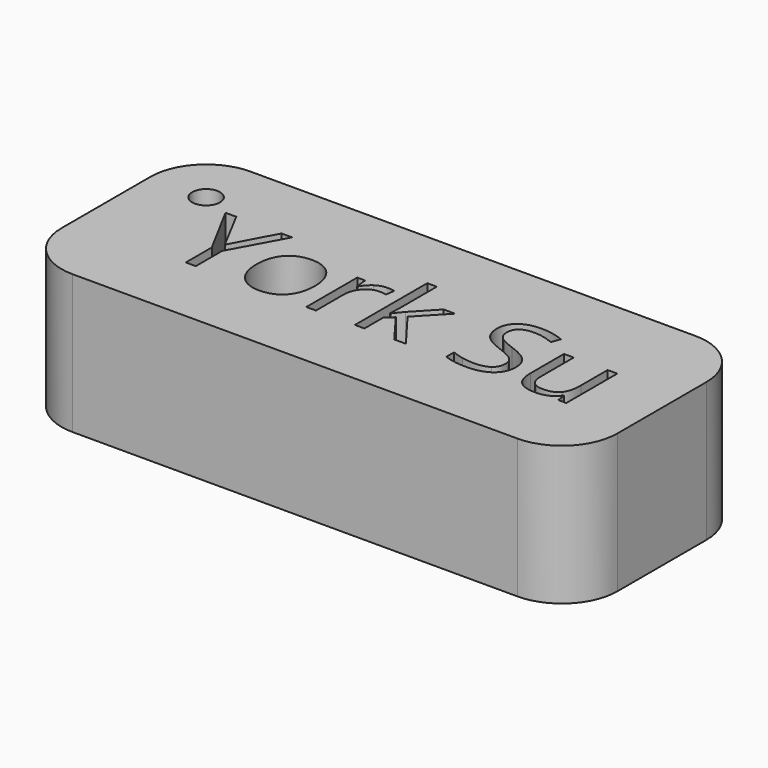
from build123d import *

# Parameters (mm, degrees)
F0_R     = 2.5
F1_DEPTH = 25


with BuildPart() as f1:
    # F0 (on Top) → F1 (new body)
    with BuildSketch(Plane.XY):
        with BuildLine():
            Line((90, 37.539282998), (10, 37.539282998))
            ThreePointArc((10, 37.539282998), (2.9289321881, 34.6103508099), (0, 27.539282998))
            Line((0, 27.539282998), (0, 7.539282998))
            ThreePointArc((0, 7.539282998), (2.9289321881, 0.4682151861), (10, -2.460717002))
            Line((10, -2.460717002), (90, -2.460717002))
            ThreePointArc((90, -2.460717002), (97.0710678119, 0.4682151861), (100, 7.539282998))
            Line((100, 7.539282998), (100, 27.539282998))
            ThreePointArc((100, 27.539282998), (97.0710678119, 34.6103508099), (90, 37.539282998))
        make_face()
        with BuildLine():
            add(Edge.make_bspline(
                [(37.3762699946, 20.3398448807), (38.7935582809, 18.7384931806), (38.7935582809, 16.0110080489)],
                knots=[0, 0, 0, 1, 1, 1], degree=2))
            add(Edge.make_bspline(
                [(38.7935582809, 16.0110080489), (38.7935582809, 13.2065509441), (37.3829632097, 11.6319721042)],
                knots=[0, 0, 0, 1, 1, 1], degree=2))
            add(Edge.make_bspline(
                [(37.3829632097, 11.6319721042), (35.9723681385, 10.0573932643), (33.4824921409, 10.0573932643)],
                knots=[0, 0, 0, 1, 1, 1], degree=2))
            add(Edge.make_bspline(
                [(33.4824921409, 10.0573932643), (31.94305268, 10.0573932643), (30.7516604016, 10.7802604894)],
                knots=[0, 0, 0, 1, 1, 1], degree=2))
            add(Edge.make_bspline(
                [(30.7516604016, 10.7802604894), (29.5602681232, 11.5031277145), (28.9110262636, 12.8518105466)],
                knots=[0, 0, 0, 1, 1, 1], degree=2))
            add(Edge.make_bspline(
                [(28.9110262636, 12.8518105466), (28.261784404, 14.2004933786), (28.261784404, 16.0110080489)],
                knots=[0, 0, 0, 1, 1, 1], degree=2))
            add(Edge.make_bspline(
                [(28.261784404, 16.0110080489), (28.261784404, 18.8121185462), (29.6640129564, 20.3766575635)],
                knots=[0, 0, 0, 1, 1, 1], degree=2))
            add(Edge.make_bspline(
                [(29.6640129564, 20.3766575635), (31.0662415088, 21.9411965808), (33.5561175064, 21.9411965808)],
                knots=[0, 0, 0, 1, 1, 1], degree=2))
            add(Edge.make_bspline(
                [(33.5561175064, 21.9411965808), (35.9589817084, 21.9411965808), (37.3762699946, 20.3398448807)],
                knots=[0, 0, 0, 1, 1, 1], degree=2))
        make_face(mode=Mode.SUBTRACT)
        with BuildLine():
            add(Edge.make_bspline(
                [(45.0918736404, 21.3337873152), (45.9921110642, 21.9411965808), (47.0697186868, 21.9411965808)],
                knots=[0, 0, 0, 1, 1, 1], degree=2))
            add(Edge.make_bspline(
                [(47.0697186868, 21.9411965808), (47.8327452022, 21.9411965808), (48.438481164, 21.8140254949)],
                knots=[0, 0, 0, 1, 1, 1], degree=2))
            Line((48.438481164, 21.8140254949), (48.1975254223, 20.204307276))
            add(Edge.make_bspline(
                [(48.1975254223, 20.204307276), (47.4880446273, 20.3615978296), (46.9425476009, 20.3615978296)],
                knots=[0, 0, 0, 1, 1, 1], degree=2))
            add(Edge.make_bspline(
                [(46.9425476009, 20.3615978296), (45.5503588711, 20.3615978296), (44.5631096516, 19.2321177904)],
                knots=[0, 0, 0, 1, 1, 1], degree=2))
            add(Edge.make_bspline(
                [(44.5631096516, 19.2321177904), (43.5758604322, 18.1026377512), (43.5758604322, 16.4192941668)],
                knots=[0, 0, 0, 1, 1, 1], degree=2))
            Line((43.5758604322, 16.4192941668), (43.5758604322, 10.2682295383))
            Line((43.5758604322, 10.2682295383), (41.8389711274, 10.2682295383))
            Line((41.8389711274, 10.2682295383), (41.8389711274, 21.7303603068))
            Line((41.8389711274, 21.7303603068), (43.2713191475, 21.7303603068))
            Line((43.2713191475, 21.7303603068), (43.4721155989, 19.6086111368))
            Line((43.4721155989, 19.6086111368), (43.555780787, 19.6086111368))
            add(Edge.make_bspline(
                [(43.555780787, 19.6086111368), (44.1916362165, 20.7263780497), (45.0918736404, 21.3337873152)],
                knots=[0, 0, 0, 1, 1, 1], degree=2))
        make_face(mode=Mode.SUBTRACT)
        with BuildLine():
            Line((79.0231273225, 21.7303603068), (80.7800962724, 21.7303603068))
            Line((80.7800962724, 21.7303603068), (80.7800962724, 14.2941983893))
            add(Edge.make_bspline(
                [(80.7800962724, 14.2941983893), (80.7800962724, 12.8919698369), (81.4176250056, 12.202568687)],
                knots=[0, 0, 0, 1, 1, 1], degree=2))
            add(Edge.make_bspline(
                [(81.4176250056, 12.202568687), (82.0551537389, 11.5131675371), (83.4138763935, 11.5131675371)],
                knots=[0, 0, 0, 1, 1, 1], degree=2))
            add(Edge.make_bspline(
                [(83.4138763935, 11.5131675371), (85.2143512412, 11.5131675371), (86.0443099071, 12.4953968453)],
                knots=[0, 0, 0, 1, 1, 1], degree=2))
            add(Edge.make_bspline(
                [(86.0443099071, 12.4953968453), (86.8742685729, 13.4776261535), (86.8742685729, 15.7064667642)],
                knots=[0, 0, 0, 1, 1, 1], degree=2))
            Line((86.8742685729, 15.7064667642), (86.8742685729, 21.7303603068))
            Line((86.8742685729, 21.7303603068), (88.6111578777, 21.7303603068))
            Line((88.6111578777, 21.7303603068), (88.6111578777, 10.2682295383))
            Line((88.6111578777, 10.2682295383), (87.1788098576, 10.2682295383))
            Line((87.1788098576, 10.2682295383), (86.9278142933, 11.8043223917))
            Line((86.9278142933, 11.8043223917), (86.8341092826, 11.8043223917))
            add(Edge.make_bspline(
                [(86.8341092826, 11.8043223917), (86.3019986864, 10.9576306882), (85.3549087572, 10.5075119763)],
                knots=[0, 0, 0, 1, 1, 1], degree=2))
            add(Edge.make_bspline(
                [(85.3549087572, 10.5075119763), (84.407818828, 10.0573932643), (83.1930002969, 10.0573932643)],
                knots=[0, 0, 0, 1, 1, 1], degree=2))
            add(Edge.make_bspline(
                [(83.1930002969, 10.0573932643), (81.1013705947, 10.0573932643), (80.0622489586, 11.0513356989)],
                knots=[0, 0, 0, 1, 1, 1], degree=2))
            add(Edge.make_bspline(
                [(80.0622489586, 11.0513356989), (79.0231273225, 12.0452781334), (79.0231273225, 14.2306128463)],
                knots=[0, 0, 0, 1, 1, 1], degree=2))
            Line((79.0231273225, 14.2306128463), (79.0231273225, 21.7303603068))
        make_face(mode=Mode.SUBTRACT)
        Polygon((17.0104899096, 25.5588793138), (21.0598850132, 17.9118811223), (25.1360529769, 25.5588793138), (27.060352303, 25.5588793138), (21.9567758295, 16.1984180702), (21.9567758295, 10.2682295383), (20.1596475893, 10.2682295383), (20.1596475893, 16.1147528821), (15.0661109383, 25.5588793138), align=None, mode=Mode.SUBTRACT)
        with Locations((10, 27.539282998)):
            Circle(F0_R, mode=Mode.SUBTRACT)
        with BuildLine():
            Line((52.2168010582, 16.1348325273), (52.3004662463, 16.1348325273))
            add(Edge.make_bspline(
                [(52.3004662463, 16.1348325273), (52.7489116544, 16.7740345643), (53.6692287234, 17.8081362891)],
                knots=[0, 0, 0, 1, 1, 1], degree=2))
            Line((53.6692287234, 17.8081362891), (57.3705766446, 21.7303603068))
            Line((57.3705766446, 21.7303603068), (59.4320868791, 21.7303603068))
            Line((59.4320868791, 21.7303603068), (54.7869956363, 16.8476599298))
            Line((54.7869956363, 16.8476599298), (59.7567078089, 10.2682295383))
            Line((59.7567078089, 10.2682295383), (57.6550382841, 10.2682295383))
            Line((57.6550382841, 10.2682295383), (53.6056431805, 15.6863871191))
            Line((53.6056431805, 15.6863871191), (52.3004662463, 14.5552337761))
            Line((52.3004662463, 14.5552337761), (52.3004662463, 10.2682295383))
            Line((52.3004662463, 10.2682295383), (50.5836565867, 10.2682295383))
            Line((50.5836565867, 10.2682295383), (50.5836565867, 26.5427819258))
            Line((50.5836565867, 26.5427819258), (52.3004662463, 26.5427819258))
            Line((52.3004662463, 26.5427819258), (52.3004662463, 17.9118811223))
            add(Edge.make_bspline(
                [(52.3004662463, 17.9118811223), (52.3004662463, 17.3396112358), (52.2168010582, 16.1348325273)],
                knots=[0, 0, 0, 1, 1, 1], degree=2))
        make_face(mode=Mode.SUBTRACT)
        with BuildLine():
            add(Edge.make_bspline(
                [(75.3753251217, 16.8878192201), (76.2789091531, 15.9039166081), (76.2789091531, 14.3377042871)],
                knots=[0, 0, 0, 1, 1, 1], degree=2))
            add(Edge.make_bspline(
                [(76.2789091531, 14.3377042871), (76.2789091531, 12.3196999503), (74.8147683615, 11.1885466073)],
                knots=[0, 0, 0, 1, 1, 1], degree=2))
            add(Edge.make_bspline(
                [(74.8147683615, 11.1885466073), (73.3506275699, 10.0573932643), (70.8406719272, 10.0573932643)],
                knots=[0, 0, 0, 1, 1, 1], degree=2))
            add(Edge.make_bspline(
                [(70.8406719272, 10.0573932643), (68.123226618, 10.0573932643), (66.6574125227, 10.7601808443)],
                knots=[0, 0, 0, 1, 1, 1], degree=2))
            Line((66.6574125227, 10.7601808443), (66.6574125227, 12.4736438964))
            add(Edge.make_bspline(
                [(66.6574125227, 12.4736438964), (67.6011558443, 12.0787442086), (68.7088829346, 11.8478282895)],
                knots=[0, 0, 0, 1, 1, 1], degree=2))
            add(Edge.make_bspline(
                [(68.7088829346, 11.8478282895), (69.816610025, 11.6169123704), (70.9042574702, 11.6169123704)],
                knots=[0, 0, 0, 1, 1, 1], degree=2))
            add(Edge.make_bspline(
                [(70.9042574702, 11.6169123704), (72.6813060652, 11.6169123704), (73.5815434891, 12.2912537864)],
                knots=[0, 0, 0, 1, 1, 1], degree=2))
            add(Edge.make_bspline(
                [(73.5815434891, 12.2912537864), (74.4817809129, 12.9655952024), (74.4817809129, 14.1703739109)],
                knots=[0, 0, 0, 1, 1, 1], degree=2))
            add(Edge.make_bspline(
                [(74.4817809129, 14.1703739109), (74.4817809129, 14.963519894), (74.1621798944, 15.4705309338)],
                knots=[0, 0, 0, 1, 1, 1], degree=2))
            add(Edge.make_bspline(
                [(74.1621798944, 15.4705309338), (73.8425788759, 15.9775419736), (73.0946120944, 16.4075810404)],
                knots=[0, 0, 0, 1, 1, 1], degree=2))
            add(Edge.make_bspline(
                [(73.0946120944, 16.4075810404), (72.3466453128, 16.8376201072), (70.8205922821, 17.379770526)],
                knots=[0, 0, 0, 1, 1, 1], degree=2))
            add(Edge.make_bspline(
                [(70.8205922821, 17.379770526), (68.6888032895, 18.1427970414), (67.7735061318, 19.1886118926)],
                knots=[0, 0, 0, 1, 1, 1], degree=2))
            add(Edge.make_bspline(
                [(67.7735061318, 19.1886118926), (66.8582089741, 20.2344267437), (66.8582089741, 21.9177703281)],
                knots=[0, 0, 0, 1, 1, 1], degree=2))
            add(Edge.make_bspline(
                [(66.8582089741, 21.9177703281), (66.8582089741, 23.6847791006), (68.1851388572, 24.7305939517)],
                knots=[0, 0, 0, 1, 1, 1], degree=2))
            add(Edge.make_bspline(
                [(68.1851388572, 24.7305939517), (69.5120687403, 25.7764088028), (71.7007500608, 25.7764088028)],
                knots=[0, 0, 0, 1, 1, 1], degree=2))
            add(Edge.make_bspline(
                [(71.7007500608, 25.7764088028), (73.9797897844, 25.7764088028), (75.8940492879, 24.9397569219)],
                knots=[0, 0, 0, 1, 1, 1], degree=2))
            Line((75.8940492879, 24.9397569219), (75.338512439, 23.393624246))
            add(Edge.make_bspline(
                [(75.338512439, 23.393624246), (73.4443325806, 24.1867702291), (71.657244163, 24.1867702291)],
                knots=[0, 0, 0, 1, 1, 1], degree=2))
            add(Edge.make_bspline(
                [(71.657244163, 24.1867702291), (70.244975788, 24.1867702291), (69.4501565011, 23.5810342673)],
                knots=[0, 0, 0, 1, 1, 1], degree=2))
            add(Edge.make_bspline(
                [(69.4501565011, 23.5810342673), (68.6553372143, 22.9752983056), (68.6553372143, 21.897690683)],
                knots=[0, 0, 0, 1, 1, 1], degree=2))
            add(Edge.make_bspline(
                [(68.6553372143, 21.897690683), (68.6553372143, 21.1045446998), (68.9481653726, 20.5958603563)],
                knots=[0, 0, 0, 1, 1, 1], degree=2))
            add(Edge.make_bspline(
                [(68.9481653726, 20.5958603563), (69.2409935309, 20.0871760127), (69.9370878958, 19.6638301609)],
                knots=[0, 0, 0, 1, 1, 1], degree=2))
            add(Edge.make_bspline(
                [(69.9370878958, 19.6638301609), (70.6331822607, 19.2404843092), (72.0655302809, 18.7284533581)],
                knots=[0, 0, 0, 1, 1, 1], degree=2))
            add(Edge.make_bspline(
                [(72.0655302809, 18.7284533581), (74.4717410903, 17.871721832), (75.3753251217, 16.8878192201)],
                knots=[0, 0, 0, 1, 1, 1], degree=2))
        make_face(mode=Mode.SUBTRACT)
    extrude(amount=F1_DEPTH)


solid = f1.part
